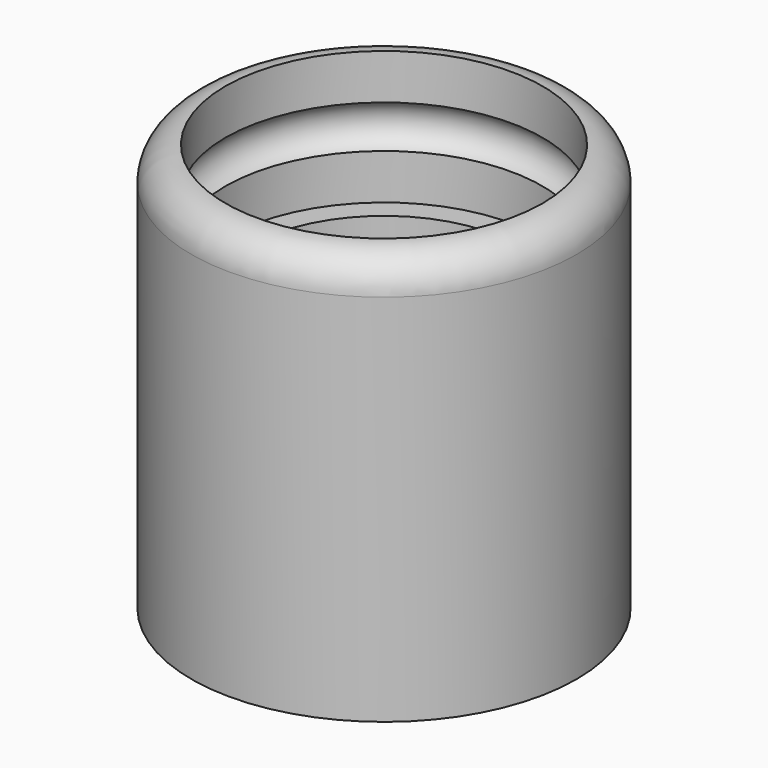
from build123d import *

# Parameters (mm, degrees)
F2_R     = 1.49999
F4_R     = 2.5
F5_DEPTH = 25


# Not quite as in the source:
# - a fillet or chamfer is up to 0.001 mm smaller than in the source, because OpenCascade refuses the exact size


with BuildPart() as f1:
    # F0 (on Front) → F1 (revolve)
    with BuildSketch(Plane.XZ):
        with BuildLine():
            Line((-29.2452627023, 12.6545929811), (-30.7452627023, 12.6545929811))
            Line((-30.7452627023, 12.6545929811), (-30.7452627023, -5.3454070189))
            Line((-30.7452627023, -5.3454070189), (-28.2452627023, -5.3454070189))
            Line((-28.2452627023, -5.3454070189), (-28.2452627023, 6.7686133647))
            Line((-28.2452627023, 6.7686133647), (-29.2452627023, 6.7686133647))
            Line((-29.2452627023, 6.7686133647), (-29.2452627023, 8.7686133647))
            ThreePointArc((-29.2452627023, 8.7686133647), (-29.9124410959, 9.7116031729), (-29.2452627023, 10.6545929811))
            Line((-29.2452627023, 10.6545929811), (-29.2452627023, 12.6545929811))
        make_face()
    revolve(axis=Axis((-22.2452627023, 0, 3.276667092), (0, 0, -1)))

    # F2 (radius 1.5 in the source; OpenCascade refuses exactly that, so slightly less here)
    f2_edges = [f1.edges().sort_by_distance(p)[0] for p in [
        (-13.745263, 0, 12.654593),
    ]]
    fillet(f2_edges, radius=F2_R)

    # F4 (on offset) → F5 (cut)
    with BuildSketch(Plane.YZ.offset(-25)):
        with Locations((0, -4.6502733603)):
            Circle(F4_R)
    extrude(amount=-F5_DEPTH, mode=Mode.SUBTRACT)


solid = f1.part
